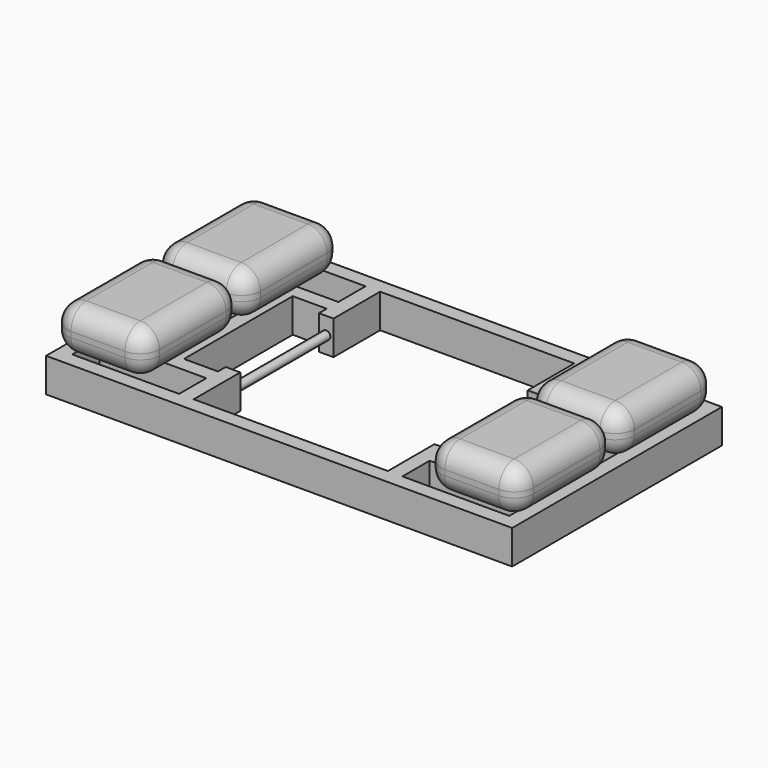
from build123d import *

# Parameters (mm, degrees)
F0_W     = 1219.2
F0_H     = 685.8
F0_W_2   = 152.4
F0_H_2   = 38.1
F1_DEPTH = 44.45
F3_W     = 241.3
F3_H     = 317.5
F4_DEPTH = 114.3
F5_R     = 50
F5_2_R   = 50
F5_3_R   = 50
F5_4_R   = 50
F6_R     = 11.049
F7_DEPTH = 228.6


# Not quite as in the source:
# - a feature names something its author has since deleted; it is built from what else it names


with BuildPart() as f1:
    # F0 (on Top) → F1 (new body, symmetric)
    with BuildSketch(Plane.XY):
        Rectangle(F0_W, F0_H)
        Polygon((292.1, 304.8), (571.5, 304.8), (571.5, 215.9), (571.5, 177.8), (571.5, 88.9), (571.5, 50.8), (571.5, -50.8), (571.5, -88.9), (571.5, -177.8), (571.5, -215.9), (571.5, -304.8), (292.1, -304.8), (254, -304.8), (-254, -304.8), (-292.1, -304.8), (-571.5, -304.8), (-571.5, -215.9), (-571.5, -177.8), (-571.5, -88.9), (-571.5, -50.8), (-571.5, 50.8), (-571.5, 88.9), (-571.5, 177.8), (-571.5, 215.9), (-571.5, 304.8), (-292.1, 304.8), (-254, 304.8), (254, 304.8), align=None, mode=Mode.SUBTRACT)
        Polygon((-292.1, -177.8), (-381, -177.8), (-419.1, -177.8), (-571.5, -177.8), (-571.5, -215.9), (-292.1, -215.9), align=None)
        with Locations((-495.3, -69.85)):
            Rectangle(F0_W_2, F0_H_2)
        with Locations((-495.3, 69.85)):
            Rectangle(F0_W_2, F0_H_2)
        Polygon((-292.1, 177.8), (-292.1, 215.9), (-571.5, 215.9), (-571.5, 177.8), (-419.1, 177.8), (-381, 177.8), align=None)
        Polygon((571.5, 177.8), (571.5, 215.9), (292.1, 215.9), (292.1, 177.8), (381, 177.8), (419.1, 177.8), align=None)
        with Locations((495.3, 69.85)):
            Rectangle(F0_W_2, F0_H_2)
        with Locations((495.3, -69.85)):
            Rectangle(F0_W_2, F0_H_2)
        Polygon((419.1, -177.8), (381, -177.8), (292.1, -177.8), (292.1, -215.9), (571.5, -215.9), (571.5, -177.8), align=None)
        Polygon((-381, -177.8), (-381, 177.8), (-419.1, 177.8), (-419.1, 88.9), (-419.1, 50.8), (-419.1, -50.8), (-419.1, -88.9), (-419.1, -177.8), align=None)
        Polygon((-254, 152.4), (-254, 304.8), (-292.1, 304.8), (-292.1, 215.9), (-292.1, 177.8), (-292.1, 152.4), align=None)
        Polygon((-292.1, -152.4), (-292.1, -177.8), (-292.1, -215.9), (-292.1, -304.8), (-254, -304.8), (-254, -152.4), align=None)
        Polygon((292.1, -215.9), (292.1, -177.8), (292.1, -152.4), (254, -152.4), (254, -304.8), (292.1, -304.8), align=None)
        Polygon((292.1, 215.9), (292.1, 304.8), (254, 304.8), (254, 152.4), (292.1, 152.4), (292.1, 177.8), align=None)
        Polygon((419.1, 88.9), (419.1, 177.8), (381, 177.8), (381, -177.8), (419.1, -177.8), (419.1, -88.9), (419.1, -50.8), (419.1, 50.8), align=None)
    extrude(amount=F1_DEPTH, both=True)


with BuildPart() as f4:
    # F3 (on offset) → F4 (new body)
    with BuildSketch(Plane.XY.offset(44.95)):
        with Locations((488.95, 165.1)):
            Rectangle(F3_W, F3_H)
    extrude(amount=F4_DEPTH)

    # F5#4
    f5_4_edges = [f4.edges().sort_by_distance(p)[0] for p in [
        (609.6, 165.1, 159.25),
        (488.95, 323.85, 159.25),
        (368.3, 165.1, 159.25),
        (488.95, 6.35, 159.25),
        (368.3, 323.85, 102.1),
        (368.3, 6.35, 102.1),
        (368.3, 165.1, 44.95),
        (609.6, 6.35, 102.1),
        (609.6, 323.85, 102.1),
        (609.6, 165.1, 44.95),
        (488.95, 323.85, 44.95),
        (488.95, 6.35, 44.95),
    ]]
    fillet(f5_4_edges, radius=F5_4_R)


with BuildPart() as f4b:
    # F3 (on offset) → F4, piece 2 (new body)
    with BuildSketch(Plane.XY.offset(44.95)):
        with Locations((488.95, -165.1)):
            Rectangle(F3_W, F3_H)
    extrude(amount=F4_DEPTH)

    # F5#3
    f5_3_edges = [f4b.edges().sort_by_distance(p)[0] for p in [
        (609.6, -165.1, 159.25),
        (488.95, -6.35, 159.25),
        (368.3, -165.1, 159.25),
        (488.95, -323.85, 159.25),
        (368.3, -6.35, 102.1),
        (368.3, -323.85, 102.1),
        (368.3, -165.1, 44.95),
        (609.6, -323.85, 102.1),
        (609.6, -6.35, 102.1),
        (609.6, -165.1, 44.95),
        (488.95, -6.35, 44.95),
        (488.95, -323.85, 44.95),
    ]]
    fillet(f5_3_edges, radius=F5_3_R)


with BuildPart() as f4c:
    # F3 (on offset) → F4, piece 3 (new body)
    with BuildSketch(Plane.XY.offset(44.95)):
        with Locations((-488.95, -165.1)):
            Rectangle(F3_W, F3_H)
    extrude(amount=F4_DEPTH)

    # F5#2
    f5_2_edges = [f4c.edges().sort_by_distance(p)[0] for p in [
        (-609.6, -165.1, 159.25),
        (-488.95, -323.85, 159.25),
        (-368.3, -165.1, 159.25),
        (-488.95, -6.35, 159.25),
        (-609.6, -6.35, 102.1),
        (-609.6, -323.85, 102.1),
        (-609.6, -165.1, 44.95),
        (-368.3, -323.85, 102.1),
        (-368.3, -6.35, 102.1),
        (-368.3, -165.1, 44.95),
        (-488.95, -323.85, 44.95),
        (-488.95, -6.35, 44.95),
    ]]
    fillet(f5_2_edges, radius=F5_2_R)


with BuildPart() as f4d:
    # F3 (on offset) → F4, piece 4 (new body)
    with BuildSketch(Plane.XY.offset(44.95)):
        with Locations((-488.95, 165.1)):
            Rectangle(F3_W, F3_H)
    extrude(amount=F4_DEPTH)

    # F5
    f5_edges = [f4d.edges().sort_by_distance(p)[0] for p in [
        (-368.3, 165.1, 159.25),
        (-488.95, 323.85, 159.25),
        (-609.6, 165.1, 159.25),
        (-488.95, 6.35, 159.25),
        (-609.6, 323.85, 102.1),
        (-609.6, 6.35, 102.1),
        (-609.6, 165.1, 44.95),
        (-368.3, 165.1, 44.95),
        (-488.95, 323.85, 44.95),
        (-488.95, 6.35, 44.95),
        (-368.3, 6.35, 102.1),
        (-368.3, 323.85, 102.1),
    ]]
    fillet(f5_edges, radius=F5_R)


with BuildPart() as f7:
    # F6 (on Front) → F7 (new body, symmetric)
    with BuildSketch(Plane.XZ):
        with Locations((-273.05, 0)):
            Circle(F6_R)
    extrude(amount=F7_DEPTH, both=True)


with BuildPart() as f7b:
    # F6 (on Front) → F7, piece 2 (new body, symmetric)
    with BuildSketch(Plane.XZ):
        with Locations((273.05, 0)):
            Circle(F6_R)
    extrude(amount=F7_DEPTH, both=True)


solid = Compound([f1.part, f4.part, f4b.part, f4c.part, f4d.part, f7.part, f7b.part])
